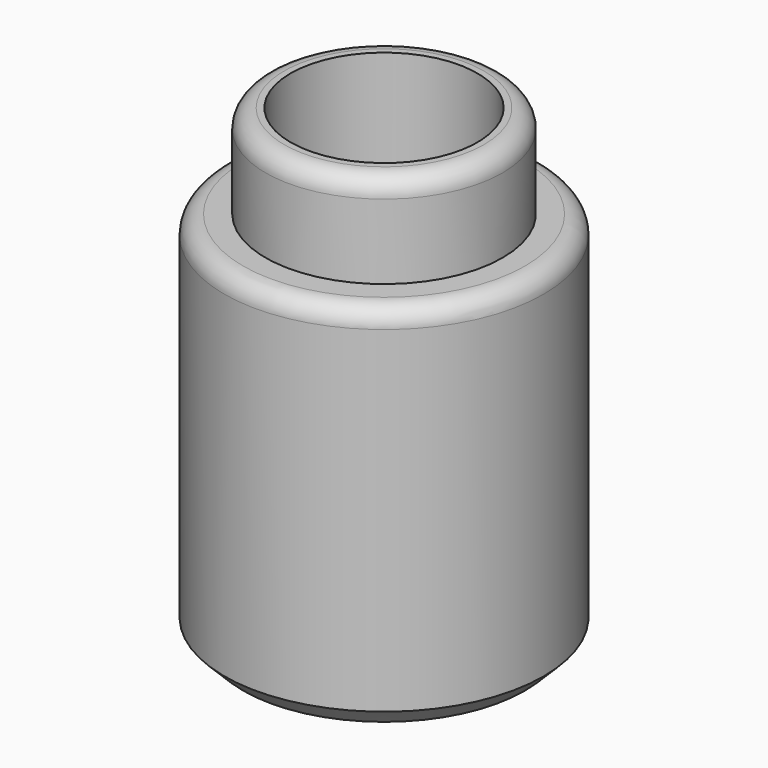
from build123d import *

# Parameters (mm, degrees)
F0_R      = 43.406760719
F0_R_2    = 31.872207378
F1_DEPTH  = 101.6
F2_R      = 32.2297053781
F3_DEPTH  = 127
F4_R      = 21.0037337021
F5_DEPTH  = 132.08
F6_R      = 5.07999
F7_SIZE   = 5.08
F9_D      = 50.8
F10_R     = 25.396952853
F11_DEPTH = 2.54


# Not quite as in the source:
# - a fillet or chamfer is up to 0.001 mm smaller than in the source, because OpenCascade refuses the exact size


with BuildPart() as f1:
    # F0 (on Top) → F1 (new body)
    with BuildSketch(Plane.XY):
        Circle(F0_R)
        Circle(F0_R_2, mode=Mode.SUBTRACT)
    extrude(amount=F1_DEPTH)

    # F2 (on Top) → F3 (join)
    with BuildSketch(Plane.XY):
        Circle(F2_R)
    extrude(amount=F3_DEPTH)

    # F4 (on Top) → F5 (join)
    with BuildSketch(Plane.XY):
        Circle(F4_R)
    extrude(amount=F5_DEPTH)

    # F6 (radius 5.08 in the source; OpenCascade refuses exactly that, so slightly less here)
    f6_edges = [f1.edges().sort_by_distance(p)[0] for p in [
        (-43.406761, 0, 101.6),
        (-32.229705, 0, 127),
        (-21.003734, 0, 132.08),
    ]]
    fillet(f6_edges, radius=F6_R)

    # F7
    f7_edges = [f1.edges().sort_by_distance(p)[0] for p in [
        (-43.406761, 0, 0),
    ]]
    chamfer(f7_edges, length=F7_SIZE)

    # F9 (through all)
    with Locations(Plane.XY.offset(132.08)):
        with Locations((0, 0)):
            Hole(F9_D / 2)


with BuildPart() as f11:
    # F10 (on Top) → F11 (new body)
    with BuildSketch(Plane.XY):
        Circle(F10_R)
    extrude(amount=F11_DEPTH)


solid = Compound([f1.part, f11.part])
